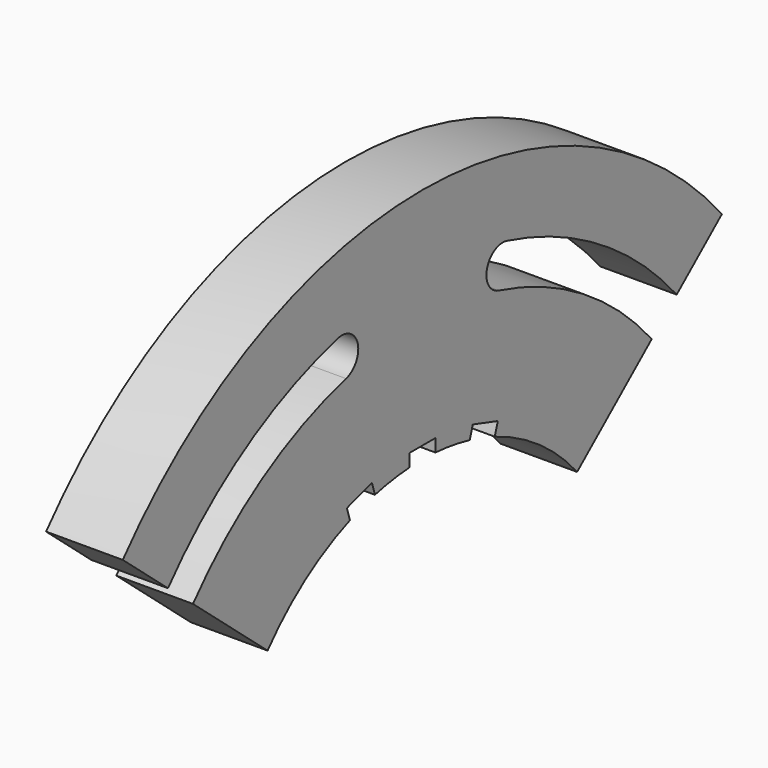
from build123d import *

# Parameters (mm, degrees)
F1_DEPTH = 3.175
F3_DEPTH = 6.35


with BuildPart() as f1:
    # F0 (on Right) → F1 (new body)
    with BuildSketch(Plane.YZ):
        with BuildLine():
            ThreePointArc((11.2416642137, 13.194756409), (18.2070674879, 9.4741128861), (24.0282094439, 4.1379778313))
            Line((24.0282094439, 4.1379778313), (35.6114845565, 13.9572464754))
            ThreePointArc((35.6114845565, 13.9572464754), (24.8807782287, 23.2715946139), (11.8451676598, 28.9265036877))
            ThreePointArc((11.8451676598, 28.9265036877), (10.0327447326, 32.0278458379), (13.1340868829, 33.8402687651))
            ThreePointArc((13.1340868829, 33.8402687651), (27.588153444, 27.5700268215), (39.4865100795, 17.2421478736))
            Line((39.4865100795, 17.2421478736), (46.5087493001, 23.1949766478))
            ThreePointArc((46.5087493001, 23.1949766478), (0, 44.7400710849), (-46.5087493001, 23.1949766478))
            Line((-46.5087493001, 23.1949766478), (-39.4865100795, 17.2421478736))
            ThreePointArc((-39.4865100795, 17.2421478736), (-27.588153444, 27.5700268215), (-13.1340868829, 33.8402687651))
            ThreePointArc((-13.1340868829, 33.8402687651), (-10.0327447326, 32.0278458379), (-11.8451676598, 28.9265036877))
            ThreePointArc((-11.8451676598, 28.9265036877), (-24.8807782287, 23.2715946139), (-35.6114845565, 13.9572464754))
            Line((-35.6114845565, 13.9572464754), (-24.0282094439, 4.1379778313))
            ThreePointArc((-24.0282094439, 4.1379778313), (-18.2070674879, 9.4741128861), (-11.2416642137, 13.194756409))
            Line((-11.2416642137, 13.194756409), (-11.7119892349, 14.7131928424))
            Line((-11.7119892349, 14.7131928424), (-7.8299477766, 15.9156279202))
            Line((-7.8299477766, 15.9156279202), (-7.3596227555, 14.3971914867))
            ThreePointArc((-7.3596227555, 14.3971914867), (-4.7130812866, 14.9144174535), (-2.032, 15.2033942376))
            Line((-2.032, 15.2033942376), (-2.032, 16.7930026258))
            Line((-2.032, 16.7930026258), (2.032, 16.7930026258))
            Line((2.032, 16.7930026258), (2.032, 15.2033942376))
            ThreePointArc((2.032, 15.2033942376), (4.7130812866, 14.9144174535), (7.3596227555, 14.3971914867))
            Line((7.3596227555, 14.3971914867), (7.8299477766, 15.9156279202))
            Line((7.8299477766, 15.9156279202), (11.7119892349, 14.7131928424))
            Line((11.7119892349, 14.7131928424), (11.2416642137, 13.194756409))
        make_face()
    extrude(amount=F1_DEPTH)

    # F2 (on face) → F3 (join)
    with BuildSketch(Plane(origin=(0, 0, 0), x_dir=(0, -1, 0), z_dir=(-1, 0, 0))):
        with BuildLine():
            Line((-2.032, 16.7930026258), (2.032, 16.7930026258))
            Line((2.032, 16.7930026258), (2.032, 15.2690026258))
            Line((2.032, 15.2690026258), (2.032, 15.2033942376))
            ThreePointArc((2.032, 15.2033942376), (4.7130812866, 14.9144174535), (7.3596227555, 14.3971914867))
            Line((7.3596227555, 14.3971914867), (7.3790346224, 14.4598623733))
            Line((7.3790346224, 14.4598623733), (7.8299477766, 15.9156279202))
            Line((7.8299477766, 15.9156279202), (11.7119892349, 14.7131928424))
            Line((11.7119892349, 14.7131928424), (11.2610760807, 13.2574272956))
            Line((11.2610760807, 13.2574272956), (11.2416642137, 13.194756409))
            ThreePointArc((11.2416642137, 13.194756409), (18.2070674879, 9.4741128861), (24.0282094439, 4.1379778313))
            Line((24.0282094439, 4.1379778313), (35.6114845565, 13.9572464754))
            ThreePointArc((35.6114845565, 13.9572464754), (24.8807782287, 23.2715946139), (11.8451676598, 28.9265036877))
            ThreePointArc((11.8451676598, 28.9265036877), (10.0327447326, 32.0278458379), (13.1340868829, 33.8402687651))
            ThreePointArc((13.1340868829, 33.8402687651), (27.588153444, 27.5700268215), (39.4865100795, 17.2421478736))
            Line((39.4865100795, 17.2421478736), (46.5087493001, 23.1949766478))
            ThreePointArc((46.5087493001, 23.1949766478), (0, 44.7400710849), (-46.5087493001, 23.1949766478))
            Line((-46.5087493001, 23.1949766478), (-39.4865100795, 17.2421478736))
            ThreePointArc((-39.4865100795, 17.2421478736), (-27.588153444, 27.5700268215), (-13.1340868829, 33.8402687651))
            ThreePointArc((-13.1340868829, 33.8402687651), (-10.0327447326, 32.0278458379), (-11.8451676598, 28.9265036877))
            ThreePointArc((-11.8451676598, 28.9265036877), (-24.8807782287, 23.2715946139), (-35.6114845565, 13.9572464754))
            Line((-35.6114845565, 13.9572464754), (-24.0282094439, 4.1379778313))
            ThreePointArc((-24.0282094439, 4.1379778313), (-18.2070674879, 9.4741128861), (-11.2416642137, 13.194756409))
            Line((-11.2416642137, 13.194756409), (-11.2610760807, 13.2574272956))
            Line((-11.2610760807, 13.2574272956), (-11.7119892349, 14.7131928424))
            Line((-11.7119892349, 14.7131928424), (-7.8299477766, 15.9156279202))
            Line((-7.8299477766, 15.9156279202), (-7.3790346224, 14.4598623733))
            Line((-7.3790346224, 14.4598623733), (-7.3596227555, 14.3971914867))
            ThreePointArc((-7.3596227555, 14.3971914867), (-4.7130812866, 14.9144174535), (-2.032, 15.2033942376))
            Line((-2.032, 15.2033942376), (-2.032, 15.2690026258))
            Line((-2.032, 15.2690026258), (-2.032, 16.7930026258))
        make_face()
    extrude(amount=F3_DEPTH)


solid = f1.part
